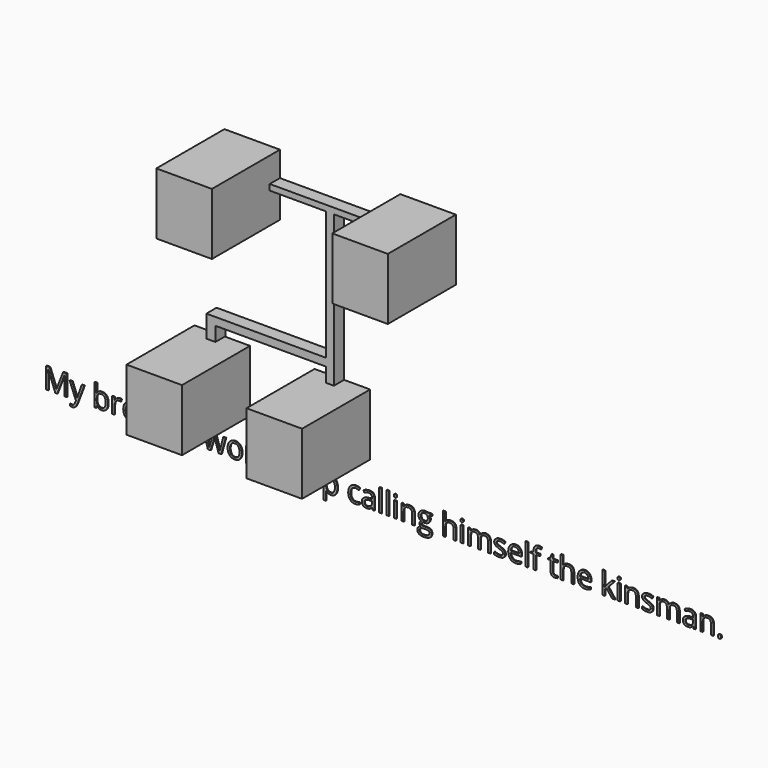
from build123d import *

# Parameters (mm, degrees)
F1_DEPTH     = 5.08
F0_W         = 3.3183861524
F0_H         = 3.687094897
F0_W_2       = 0.5425810814
F0_H_2       = 0.8526276797
F2_DEPTH     = 0.762
F3_TEXT_SIZE = 1.7419172865
F4_DEPTH     = 0.0508


# Not quite as in the source:
# - Text() gives the source's letters only with a copy of the font that has no kerning and outlines rounded to 1/6400 em; it was checked with that copy


with BuildPart() as f1:
    # F0 (on Front) → F1 (new body)
    with BuildSketch(Plane.XZ):
        Polygon((-23.4130639583, 38.5301597416), (-23.4130639583, 37.0355062187), (-23.4130639583, 36.6866122931), (-23.4130639583, 34.8430648446), (-20.0946778059, 34.8430648446), (-20.0946778059, 38.5301597416), align=None)
    extrude(amount=F1_DEPTH)


with BuildPart() as f1b:
    # F0 (on Front) → F1, piece 2 (new body)
    with BuildSketch(Plane.XZ):
        Polygon((-25.218244642, 27.6708062738), (-26.7711542547, 27.6708062738), (-27.0079839975, 27.6708062738), (-27.2448137403, 27.6708062738), (-28.5366307944, 27.6708062738), (-28.5366307944, 23.9837113768), (-25.218244642, 23.9837113768), align=None)
    extrude(amount=F1_DEPTH)


with BuildPart() as f1c:
    # F0 (on Front) → F1, piece 3 (new body)
    with BuildSketch(Plane.XZ):
        with Locations((-34.0472673997, 25.7885027677)):
            Rectangle(F0_W, F0_H)
    extrude(amount=F1_DEPTH)


with BuildPart() as f1d:
    # F0 (on Front) → F1, piece 4 (new body)
    with BuildSketch(Plane.XZ):
        Polygon((-30.6029040366, 38.5301597416), (-33.921290189, 38.5301597416), (-33.921290189, 34.8430648446), (-30.6029040366, 34.8430648446), (-30.6029040366, 36.6866122931), (-30.6029040366, 37.0355062187), align=None)
    extrude(amount=F1_DEPTH)


with BuildPart() as f2:
    # F0 (on Front) → F2 (new body)
    with BuildSketch(Plane.XZ):
        Polygon((-23.4130639583, 37.0355062187), (-30.6029040366, 37.0355062187), (-30.6029040366, 36.6866122931), (-27.2448137403, 36.6866122931), (-26.7711542547, 36.6866122931), (-23.4130639583, 36.6866122931), align=None)
        Polygon((-26.7711542547, 36.6866122931), (-27.2448137403, 36.6866122931), (-27.2448137403, 28.9885047823), (-27.2448137403, 28.5234339535), (-27.2448137403, 27.6708062738), (-27.0079839975, 27.6708062738), (-26.7711542547, 27.6708062738), align=None)
        Polygon((-27.2448137403, 28.5234339535), (-27.2448137403, 28.9885047823), (-34.3887619674, 28.9885047823), (-34.3887619674, 28.5234339535), (-33.846180886, 28.5234339535), (-32.4509702623, 28.5234339535), align=None)
        with Locations((-34.1174714267, 28.0971201137)):
            Rectangle(F0_W_2, F0_H_2)
    extrude(amount=F2_DEPTH)


with BuildPart() as f4:
    # F3 (on Front) → F4 (new body)
    with BuildSketch(Plane.XZ):
        with Locations((-44.7028540075, 21.4081220329)):
            Text('My brother wont stop calling himself the kinsman.', F3_TEXT_SIZE, font='Open Sans', text_align=(TextAlign.LEFT, TextAlign.BOTTOM))
    extrude(amount=F4_DEPTH)


solid = Compound([f1.part, f1b.part, f1c.part, f1d.part, f2.part, f4.part])
